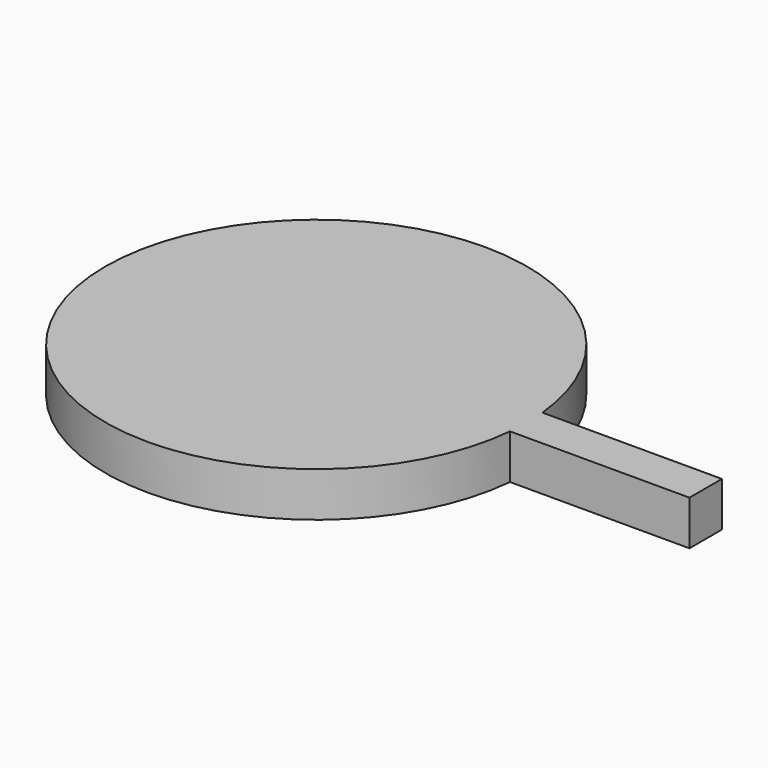
from build123d import *

# Parameters (mm, degrees)
F0_R     = 21
F1_DEPTH = 5.5
F2_DEPTH = 3


# Not quite as in the source:
# - a feature of the source that left no trace in its solid (it failed there, or was rolled back) is left out


with BuildPart() as f1:
    # F0 (on Top) → F1 (new body)
    with BuildSketch(Plane.XY):
        with BuildLine():
            ThreePointArc((25.8795285892, -2.5), (25.9698646831, -1.2514504945), (26, 0))
            ThreePointArc((26, 0), (25.9698646831, 1.2514504945), (25.8795285892, 2.5))
            ThreePointArc((25.8795285892, 2.5), (-26, 0), (25.8795285892, -2.5))
        make_face()
        Circle(F0_R, mode=Mode.SUBTRACT)
        with BuildLine():
            ThreePointArc((25.8795285892, 2.5), (25.9698646831, 1.2514504945), (26, 0))
            ThreePointArc((26, 0), (25.9698646831, -1.2514504945), (25.8795285892, -2.5))
            Line((25.8795285892, -2.5), (48, -2.5))
            Line((48, -2.5), (48, 0))
            Line((48, 0), (48, 2.5))
            Line((48, 2.5), (25.8795285892, 2.5))
        make_face()
        Circle(F0_R)
    extrude(amount=F1_DEPTH)

    # F0 (on Top) → F2 (cut)
    with BuildSketch(Plane.XY):
        Circle(F0_R)
    extrude(amount=F2_DEPTH, mode=Mode.SUBTRACT)


solid = f1.part
